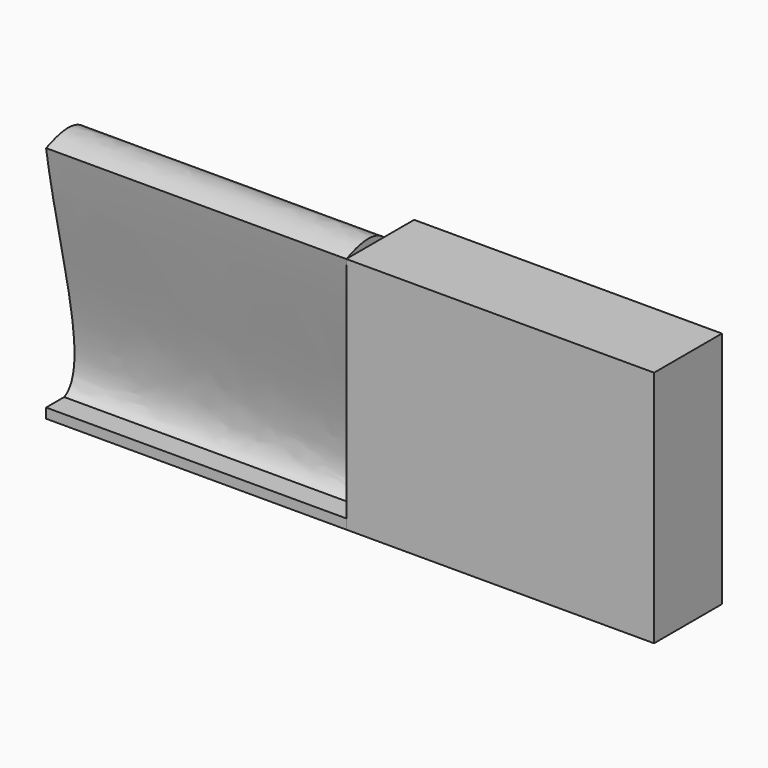
from build123d import *

# Parameters (mm, degrees)
F0_W     = 32.3
F0_H     = 8.9
F1_DEPTH = 25
F3_DEPTH = 31.5


# Not quite as in the source:
# - ends of sketch curves that miss each other by under 0.0002 mm in the source are joined
# - the dataset's text gives a spline's control points without its knots; the knots are read off the source's solid
# - a feature names something its author has since deleted; it is built from what else it names


with BuildPart() as f1:
    # F0 (on Top) → F1 (new body)
    with BuildSketch(Plane.XY):
        with Locations((5.4698575486, -0.6034393178)):
            Rectangle(F0_W, F0_H)
    extrude(amount=F1_DEPTH)


with BuildPart() as f3:
    # F2 (on face) → F3 (new body)
    with BuildSketch(Plane(origin=(-10.6801424514, 0, 0), x_dir=(0, -1, 0), z_dir=(-1, 0, 0))):
        with BuildLine():
            Line((5.0534393178, 1.0357304234), (2.6771188714, 1.0357304234))
            add(Edge.make_bspline(
                [(2.6771188714, 1.0357304234), (-0.8418467478, 2.7226619422), (3.4419558942, 14.6298892796), (5.0534393178, 25)],
                knots=[0, 0, 0, 0, 24.0818004976, 24.0818004976, 24.0818004976, 24.0818004976], degree=3))
            Line((5.0534393178, 25), (0.119884152, 25))
            add(Edge.make_bspline(
                [(0.119884152, 25), (-2.8379753894, 22.4677441836), (-2.0553450015, 13.3724585221), (-3.745077647, 1.6851037906)],
                knots=[6.6765126495, 6.6765126495, 6.6765126495, 6.6765126495, 25.2359659061, 25.2359659061, 25.2359659061, 25.2359659061], degree=3))
            add(Edge.make_bspline(
                [(-3.745077647, 1.6851037906), (-3.7779541339, 1.4577073649), (-3.8117665587, 1.2293296854), (-3.8465606822, 1)],
                knots=[25.2359659061, 25.2359659061, 25.2359659061, 25.2359659061, 25.5970701448, 25.5970701448, 25.5970701448, 25.5970701448], degree=3))
            Line((-3.8465606822, 1), (-3.8465606822, 0))
            Line((-3.8465606822, 0), (-2.3918252697, 0))
            ThreePointArc((-2.3918252697, 0), (-1.9811428085, 0.6557758803), (-1.7656583318, 1.3989235973))
            add(Edge.make_bspline(
                [(2.7973249591, 23.6349495832), (2.5542065536, 23.6832426766), (2.2182902844, 23.7171528416), (1.9025294377, 23.6958260622), (1.7187571468, 23.6535525287), (1.5872796632, 23.5988992548), (1.4682334776, 23.5245471174), (1.3331956369, 23.4054124572), (1.1209928945, 23.151165617), (0.8119295886, 22.6057356225), (0.4543623636, 21.5660702122), (0.1494819685, 20.186926591), (-0.0998810713, 18.5107135491), (-0.3750402406, 15.9253364577), (-0.6586936544, 12.1065119049), (-1.0683221986, 6.9581823178), (-1.5020900663, 3.2219080247), (-1.7656583318, 1.3989235973)],
                knots=[0.0771936817, 0.0771936817, 0.0771936817, 0.0771936817, 0.125, 0.15625, 0.1875, 0.21875, 0.25, 0.28125, 0.3125, 0.375, 0.4375, 0.5, 0.5625, 0.625, 0.75, 0.875, 0.9858927937, 0.9858927937, 0.9858927937, 0.9858927937], degree=3))
            add(Edge.make_bspline(
                [(0.742053504, 4.49535e-05), (0.6962561573, 0.0468160151), (0.4830601411, 0.2758284647), (0.1608813084, 0.7184982614), (-0.2560654542, 1.5434831509), (-0.5501272315, 2.6072939003), (-0.6855239109, 3.9304992744), (-0.6722493573, 5.3334435146), (-0.5451945541, 6.8309904438), (-0.3267180535, 8.4260370504), (0.062759398, 10.6753803152), (0.6932496185, 13.6928806547), (1.5567086755, 17.5335150811), (2.2817575639, 20.8892385574), (2.6687374058, 22.9139279094), (2.7973249591, 23.6349495832)],
                knots=[0.0542797466, 0.0542797466, 0.0542797466, 0.0542797466, 0.0625, 0.09375, 0.125, 0.1875, 0.25, 0.3125, 0.375, 0.4375, 0.5, 0.625, 0.75, 0.875, 0.9452188411, 0.9452188411, 0.9452188411, 0.9452188411], degree=3))
            Line((0.742053504, 4.49535e-05), (5.0534393178, 0))
            Line((5.0534393178, 0), (5.0534393178, 1.0357304234))
        make_face()
        with BuildLine():
            Line((0.119884152, 25), (5.0534393178, 25))
            add(Edge.make_bspline(
                [(5.0534393178, 25), (2.732042289, 25.9725657014), (1.1839341739, 25.9109448299), (0.119884152, 25)],
                knots=[0, 0, 0, 0, 6.6765126495, 6.6765126495, 6.6765126495, 6.6765126495], degree=3))
        make_face()
        with BuildLine():
            add(Edge.make_bspline(
                [(-3.745077647, 1.6851037906), (-3.7779541339, 1.4577073649), (-3.8117665587, 1.2293296854), (-3.8465606822, 1)],
                knots=[25.2359659061, 25.2359659061, 25.2359659061, 25.2359659061, 25.5970701448, 25.5970701448, 25.5970701448, 25.5970701448], degree=3))
            ThreePointArc((-3.745077647, 1.6851037906), (-3.7817745844, 1.5352780015), (-3.8465606822, 1.3952880238))
            Line((-3.8465606822, 1.3952880238), (-3.8465606822, 1))
        make_face()
        with BuildLine():
            Line((-3.8465606822, 0), (-3.8465606822, 1))
            Line((-3.8465606822, 1), (-3.8465606822, 1.3952880238))
            ThreePointArc((-3.8465606822, 1.3952880238), (-4.1388415136, 1.105825773), (-4.5363555194, 1))
            Line((-4.5363555194, 1), (-4.8465606822, 1))
            Line((-4.8465606822, 1), (-4.8465606822, 0))
            Line((-4.8465606822, 0), (-3.8465606822, 0))
        make_face()
    extrude(amount=F3_DEPTH)


solid = Compound([f1.part, f3.part])
